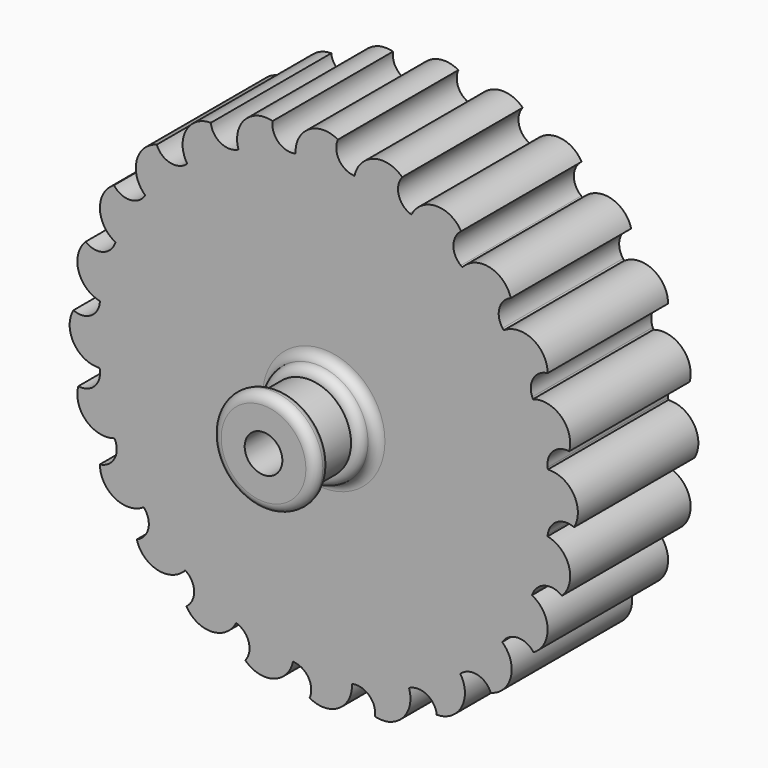
from build123d import *

# Parameters (mm, degrees)
F1_DEPTH     = 50.8
F2_R         = 17.4625
F3_DEPTH     = 6.35
F4_R         = 14.2875
F5_DEPTH     = 12.7
F6_R         = 17.4625
F7_DEPTH     = 6.35
F8_R         = 3.17499
F9_R         = 6.35
F10_DEPTH    = 76.201
F11_T1_DEPTH = 50.8


# Not quite as in the source:
# - a fillet or chamfer that OpenCascade refuses, or shapes differently, is made with other operations: its cross-section is extruded or revolved along the edge and cut away or added
# - a fillet or chamfer is up to 0.001 mm smaller than in the source, because OpenCascade refuses the exact size


with BuildPart() as f1:
    # F0 (on Front) → F1 (new body)
    with BuildSketch(Plane.XZ):
        with BuildLine():
            ThreePointArc((-70.7536357684, 46.348891971), (-75.5114792005, 37.8021981611), (-70.2287691608, 29.5695786604))
            ThreePointArc((-70.2287691608, 29.5695786604), (-72.0845164259, 24.7034914868), (-73.6035479632, 19.7220112368))
            Line((-73.6035479632, 19.7220112368), (-80.338740054, 26.4572033276))
            ThreePointArc((-80.338740054, 26.4572033276), (-82.7224167718, 16.9703105533), (-75.4889519939, 10.3854767276))
            ThreePointArc((-75.4889519939, 10.3854767276), (-76.0220301687, 5.2048947186), (-76.2, 0))
            Line((-76.2, 0), (-84.448891971, 4.7625))
            ThreePointArc((-84.448891971, 4.7625), (-84.2959583455, -5.0180756738), (-75.6046875, -9.5063782813))
            ThreePointArc((-75.6046875, -9.5063782813), (-74.7787681878, -14.6484070232), (-73.6035479632, -19.7220112368))
            Line((-73.6035479632, -19.7220112368), (-82.8039914586, -17.2567598322))
            ThreePointArc((-82.8039914586, -17.2567598322), (-80.1248696635, -26.6644883366), (-70.5680884956, -28.7503893204))
            ThreePointArc((-70.5680884956, -28.7503893204), (-68.4394567327, -33.503444034), (-65.9911357684, -38.1))
            Line((-65.9911357684, -38.1), (-75.5161357684, -38.1))
            ThreePointArc((-75.5161357684, -38.1), (-70.4934035266, -46.4937601844), (-60.7223908795, -46.0351088396))
            ThreePointArc((-60.7223908795, -46.0351088396), (-57.4361094027, -50.075276701), (-53.8815367264, -53.8815367264))
            Line((-53.8815367264, -53.8815367264), (-63.0819802218, -56.346788131))
            ThreePointArc((-63.0819802218, -56.346788131), (-56.0579284352, -63.1545591102), (-46.7385626735, -60.182611768))
            ThreePointArc((-46.7385626735, -60.182611768), (-42.5185861347, -63.234562014), (-38.1, -65.9911357684))
            Line((-38.1, -65.9911357684), (-46.348891971, -70.7536357684))
            ThreePointArc((-46.348891971, -70.7536357684), (-37.8021981611, -75.5114792005), (-29.5695786604, -70.2287691608))
            ThreePointArc((-29.5695786604, -70.2287691608), (-24.7034914868, -72.0845164259), (-19.7220112368, -73.6035479632))
            Line((-19.7220112368, -73.6035479632), (-26.4572033276, -80.338740054))
            ThreePointArc((-26.4572033276, -80.338740054), (-16.9703105533, -82.7224167718), (-10.3854767276, -75.4889519939))
            ThreePointArc((-10.3854767276, -75.4889519939), (-5.2048947186, -76.0220301687), (0, -76.2))
            Line((0, -76.2), (-4.7625, -84.448891971))
            ThreePointArc((-4.7625, -84.448891971), (5.0180756738, -84.2959583455), (9.5063782813, -75.6046875))
            ThreePointArc((9.5063782813, -75.6046875), (14.6484070232, -74.7787681878), (19.7220112368, -73.6035479632))
            Line((19.7220112368, -73.6035479632), (17.2567598322, -82.8039914586))
            ThreePointArc((17.2567598322, -82.8039914586), (26.6644883366, -80.1248696635), (28.7503893204, -70.5680884956))
            ThreePointArc((28.7503893204, -70.5680884956), (33.503444034, -68.4394567327), (38.1, -65.9911357684))
            Line((38.1, -65.9911357684), (38.1, -75.5161357684))
            ThreePointArc((38.1, -75.5161357684), (46.4937601844, -70.4934035266), (46.0351088396, -60.7223908795))
            ThreePointArc((46.0351088396, -60.7223908795), (50.075276701, -57.4361094027), (53.8815367264, -53.8815367264))
            Line((53.8815367264, -53.8815367264), (56.346788131, -63.0819802218))
            ThreePointArc((56.346788131, -63.0819802218), (63.1545591102, -56.0579284352), (60.182611768, -46.7385626735))
            ThreePointArc((60.182611768, -46.7385626735), (63.234562014, -42.5185861347), (65.9911357684, -38.1))
            Line((65.9911357684, -38.1), (70.7536357684, -46.348891971))
            ThreePointArc((70.7536357684, -46.348891971), (75.5114792005, -37.8021981611), (70.2287691608, -29.5695786604))
            ThreePointArc((70.2287691608, -29.5695786604), (72.0845164259, -24.7034914868), (73.6035479632, -19.7220112368))
            Line((73.6035479632, -19.7220112368), (80.338740054, -26.4572033276))
            ThreePointArc((80.338740054, -26.4572033276), (82.7224167718, -16.9703105533), (75.4889519939, -10.3854767276))
            ThreePointArc((75.4889519939, -10.3854767276), (76.0220301687, -5.2048947186), (76.2, 0))
            Line((76.2, 0), (84.448891971, -4.7625))
            ThreePointArc((84.448891971, -4.7625), (84.2959583455, 5.0180756738), (75.6046875, 9.5063782813))
            ThreePointArc((75.6046875, 9.5063782813), (74.7787681878, 14.6484070232), (73.6035479632, 19.7220112368))
            Line((73.6035479632, 19.7220112368), (82.8039914586, 17.2567598322))
            ThreePointArc((82.8039914586, 17.2567598322), (80.1248696635, 26.6644883366), (70.5680884956, 28.7503893204))
            ThreePointArc((70.5680884956, 28.7503893204), (68.4394567327, 33.503444034), (65.9911357684, 38.1))
            Line((65.9911357684, 38.1), (75.5161357684, 38.1))
            ThreePointArc((75.5161357684, 38.1), (70.4934035266, 46.4937601844), (60.7223908795, 46.0351088396))
            ThreePointArc((60.7223908795, 46.0351088396), (57.4361094027, 50.075276701), (53.8815367264, 53.8815367264))
            Line((53.8815367264, 53.8815367264), (63.0819802218, 56.346788131))
            ThreePointArc((63.0819802218, 56.346788131), (56.0579284352, 63.1545591102), (46.7385626735, 60.182611768))
            ThreePointArc((46.7385626735, 60.182611768), (42.5185861347, 63.234562014), (38.1, 65.9911357684))
            Line((38.1, 65.9911357684), (46.348891971, 70.7536357684))
            ThreePointArc((46.348891971, 70.7536357684), (37.8021981611, 75.5114792005), (29.5695786604, 70.2287691608))
            ThreePointArc((29.5695786604, 70.2287691608), (24.7034914868, 72.0845164259), (19.7220112368, 73.6035479632))
            Line((19.7220112368, 73.6035479632), (26.4572033276, 80.338740054))
            ThreePointArc((26.4572033276, 80.338740054), (16.9703105533, 82.7224167718), (10.3854767276, 75.4889519939))
            ThreePointArc((10.3854767276, 75.4889519939), (5.2048947186, 76.0220301687), (0, 76.2))
            Line((0, 76.2), (4.7625, 84.448891971))
            ThreePointArc((4.7625, 84.448891971), (-5.0180756738, 84.2959583455), (-9.5063782813, 75.6046875))
            ThreePointArc((-9.5063782813, 75.6046875), (-14.6484070232, 74.7787681878), (-19.7220112368, 73.6035479632))
            Line((-19.7220112368, 73.6035479632), (-17.2567598322, 82.8039914586))
            ThreePointArc((-17.2567598322, 82.8039914586), (-26.6644883366, 80.1248696635), (-28.7503893204, 70.5680884956))
            ThreePointArc((-28.7503893204, 70.5680884956), (-33.503444034, 68.4394567327), (-38.1, 65.9911357684))
            Line((-38.1, 65.9911357684), (-38.1, 75.5161357684))
            ThreePointArc((-38.1, 75.5161357684), (-46.4937601844, 70.4934035266), (-46.0351088396, 60.7223908795))
            ThreePointArc((-46.0351088396, 60.7223908795), (-50.075276701, 57.4361094027), (-53.8815367264, 53.8815367264))
            Line((-53.8815367264, 53.8815367264), (-56.346788131, 63.0819802218))
            ThreePointArc((-56.346788131, 63.0819802218), (-63.1545591102, 56.0579284352), (-60.182611768, 46.7385626735))
            ThreePointArc((-60.182611768, 46.7385626735), (-63.234562014, 42.5185861347), (-65.9911357684, 38.1))
            Line((-65.9911357684, 38.1), (-70.7536357684, 46.348891971))
        make_face()
    extrude(amount=F1_DEPTH)

    # F2 (on face) → F3 (join)
    with BuildSketch(Plane.XZ.offset(50.8)):
        Circle(F2_R)
    extrude(amount=F3_DEPTH)

    # F4 (on face) → F5 (join)
    with BuildSketch(Plane.XZ.offset(57.15)):
        Circle(F4_R)
    extrude(amount=F5_DEPTH)

    # F6 (on face) → F7 (join)
    with BuildSketch(Plane.XZ.offset(69.85)):
        Circle(F6_R)
    extrude(amount=F7_DEPTH)

    # F8 (radius 3.175 in the source; OpenCascade refuses exactly that, so slightly less here)
    f8_edges = [f1.edges().sort_by_distance(p)[0] for p in [
        (17.4625, -73.025, 0),
        (-17.4625, -69.85, 0),
        (-17.4625, -76.2, 0),
        (17.4625, -53.975, 0),
        (-17.4625, -50.8, 0),
        (-17.4625, -57.15, 0),
    ]]
    fillet(f8_edges, radius=F8_R)

    # F9 (on face) → F10 (cut, through all)
    with BuildSketch(Plane.XZ.offset(76.2)):
        Circle(F9_R)
    extrude(amount=-F10_DEPTH, mode=Mode.SUBTRACT)

    # F11: fillet of radius 6.35 on 24 edges, made by hand

    # F11_s2 → F11_t1 (join)
    with BuildSketch(Plane.XZ):
        with BuildLine():
            ThreePointArc((-46.5419900283, 60.3347591708), (-52.1337249794, 59.2481383586), (-56.346788131, 63.0819802218))
            Line((-56.346788131, 63.0819802218), (-56.4653141097, 63.0363667109))
            ThreePointArc((-56.4653141097, 63.0363667109), (-55.2368350087, 58.4488884554), (-54.0042093064, 53.8486667077))
            Line((-54.0042093064, 53.8486667077), (-53.7917341652, 53.7917341652))
            ThreePointArc((-53.7917341652, 53.7917341652), (-50.2314688194, 57.1305598542), (-46.4644200449, 60.2342012389))
            Line((-46.4644200449, 60.2342012389), (-46.5419900283, 60.3347591708))
        make_face()
        with BuildLine():
            ThreePointArc((-29.3403254202, 70.3248555223), (-35.0227647841, 70.7225079169), (-38.1, 75.5161357684))
            Line((-38.1, 75.5161357684), (-38.2262929492, 75.5027532808))
            ThreePointArc((-38.2262929492, 75.5027532808), (-38.227, 70.7536357684), (-38.227, 65.9911357684))
            Line((-38.227, 65.9911357684), (-38.0365, 65.8811505421))
            ThreePointArc((-38.0365, 65.8811505421), (-33.7333960774, 68.1847440274), (-29.2914248778, 70.2076474298))
            Line((-29.2914248778, 70.2076474298), (-29.3403254202, 70.3248555223))
        make_face()
        with BuildLine():
            ThreePointArc((-17.2567598322, 82.8039914586), (-15.5250610467, 77.3772554351), (-10.1391661218, 75.5224291873))
            Line((-10.1391661218, 75.5224291873), (-10.1222675116, 75.396558472))
            ThreePointArc((-10.1222675116, 75.396558472), (-14.9364481399, 74.5922505758), (-19.6891412181, 73.4808753833))
            Line((-19.6891412181, 73.4808753833), (-19.8446838168, 73.636417982))
            ThreePointArc((-19.8446838168, 73.636417982), (-18.6120581145, 78.2366397297), (-17.3822130962, 82.8237519887))
            Line((-17.3822130962, 82.8237519887), (-17.2567598322, 82.8039914586))
        make_face()
        with BuildLine():
            ThreePointArc((4.7625, 84.448891971), (5.0306499446, 78.7588708674), (9.752960592, 75.5732741099))
            Line((9.752960592, 75.5732741099), (9.7367056577, 75.4473186531))
            ThreePointArc((9.7367056577, 75.4473186531), (4.8783940547, 75.916418517), (0, 76.073))
            Line((0, 76.073), (-0.1099852263, 76.2635))
            ThreePointArc((-0.1099852263, 76.2635), (2.2712647737, 80.3879459855), (4.6464358538, 84.5004488714))
            Line((4.6464358538, 84.5004488714), (4.7625, 84.448891971))
        make_face()
        with BuildLine():
            ThreePointArc((26.4572033276, 80.338740054), (25.2435304558, 74.7731994053), (28.980439159, 70.4739252926))
            Line((28.980439159, 70.4739252926), (28.9321384271, 70.3564687505))
            ThreePointArc((28.9321384271, 70.3564687505), (24.3607817564, 72.0670079941), (19.6891412181, 73.4808753833))
            Line((19.6891412181, 73.4808753833), (19.6322086756, 73.6933505244))
            ThreePointArc((19.6322086756, 73.6933505244), (22.999804721, 77.0609465698), (26.3584378791, 80.4185798071))
            Line((26.3584378791, 80.4185798071), (26.4572033276, 80.338740054))
        make_face()
        with BuildLine():
            ThreePointArc((46.348891971, 70.7536357684), (43.7361060833, 65.6918579723), (46.2329486897, 60.5718949303))
            Line((46.2329486897, 60.5718949303), (46.1558937753, 60.4709417721))
            ThreePointArc((46.1558937753, 60.4709417721), (42.1830224396, 63.3063499727), (38.0365, 65.8811505421))
            Line((38.0365, 65.8811505421), (38.0365, 66.1011209947))
            ThreePointArc((38.0365, 66.1011209947), (42.1609459855, 68.4823709947), (46.2741559222, 70.8563174269))
            Line((46.2741559222, 70.8563174269), (46.348891971, 70.7536357684))
        make_face()
        with BuildLine():
            ThreePointArc((63.0819802218, 56.346788131), (59.2481383586, 52.1337249794), (60.3347591708, 46.5419900283))
            Line((60.3347591708, 46.5419900283), (60.2342012389, 46.4644200449))
            ThreePointArc((60.2342012389, 46.4644200449), (57.1305598542, 50.2314688194), (53.7917341652, 53.7917341652))
            Line((53.7917341652, 53.7917341652), (53.8486667077, 54.0042093064))
            ThreePointArc((53.8486667077, 54.0042093064), (58.4488884554, 55.2368350087), (63.0363667109, 56.4653141097))
            Line((63.0363667109, 56.4653141097), (63.0819802218, 56.346788131))
        make_face()
        with BuildLine():
            ThreePointArc((75.5161357684, 38.1), (70.7225079169, 35.0227647841), (70.3248555223, 29.3403254202))
            Line((70.3248555223, 29.3403254202), (70.2076474298, 29.2914248778))
            ThreePointArc((70.2076474298, 29.2914248778), (68.1847440274, 33.7333960774), (65.8811505421, 38.0365))
            Line((65.8811505421, 38.0365), (65.9911357684, 38.227))
            ThreePointArc((65.9911357684, 38.227), (70.7536357684, 38.227), (75.5027532808, 38.2262929492))
            Line((75.5027532808, 38.2262929492), (75.5161357684, 38.1))
        make_face()
        with BuildLine():
            ThreePointArc((82.8039914586, 17.2567598322), (77.3772554351, 15.5250610467), (75.5224291873, 10.1391661218))
            Line((75.5224291873, 10.1391661218), (75.396558472, 10.1222675116))
            ThreePointArc((75.396558472, 10.1222675116), (74.5922505758, 14.9364481399), (73.4808753833, 19.6891412181))
            Line((73.4808753833, 19.6891412181), (73.636417982, 19.8446838168))
            ThreePointArc((73.636417982, 19.8446838168), (78.2366397297, 18.6120581144), (82.8237519887, 17.3822130962))
            Line((82.8237519887, 17.3822130962), (82.8039914586, 17.2567598322))
        make_face()
        with BuildLine():
            ThreePointArc((84.448891971, -4.7625), (78.7588708674, -5.0306499446), (75.5732741099, -9.752960592))
            Line((75.5732741099, -9.752960592), (75.4473186531, -9.7367056577))
            ThreePointArc((75.4473186531, -9.7367056577), (75.916418517, -4.8783940547), (76.073, 0))
            Line((76.073, 0), (76.2635, 0.1099852263))
            ThreePointArc((76.2635, 0.1099852263), (80.3879459855, -2.2712647737), (84.5004488714, -4.6464358538))
            Line((84.5004488714, -4.6464358538), (84.448891971, -4.7625))
        make_face()
        with BuildLine():
            ThreePointArc((80.338740054, -26.4572033276), (74.7731994053, -25.2435304558), (70.4739252926, -28.980439159))
            Line((70.4739252926, -28.980439159), (70.3564687505, -28.9321384271))
            ThreePointArc((70.3564687505, -28.9321384271), (72.0670079941, -24.3607817564), (73.4808753833, -19.6891412181))
            Line((73.4808753833, -19.6891412181), (73.6933505244, -19.6322086756))
            ThreePointArc((73.6933505244, -19.6322086756), (77.0609465698, -22.999804721), (80.4185798071, -26.3584378791))
            Line((80.4185798071, -26.3584378791), (80.338740054, -26.4572033276))
        make_face()
        with BuildLine():
            ThreePointArc((70.7536357684, -46.348891971), (65.6918579723, -43.7361060833), (60.5718949303, -46.2329486897))
            Line((60.5718949303, -46.2329486897), (60.4709417721, -46.1558937753))
            ThreePointArc((60.4709417721, -46.1558937753), (63.3063499727, -42.1830224396), (65.8811505421, -38.0365))
            Line((65.8811505421, -38.0365), (66.1011209947, -38.0365))
            ThreePointArc((66.1011209947, -38.0365), (68.4823709947, -42.1609459855), (70.8563174269, -46.2741559222))
            Line((70.8563174269, -46.2741559222), (70.7536357684, -46.348891971))
        make_face()
        with BuildLine():
            ThreePointArc((56.346788131, -63.0819802218), (52.1337249794, -59.2481383586), (46.5419900283, -60.3347591708))
            Line((46.5419900283, -60.3347591708), (46.4644200449, -60.2342012389))
            ThreePointArc((46.4644200449, -60.2342012389), (50.2314688194, -57.1305598542), (53.7917341652, -53.7917341652))
            Line((53.7917341652, -53.7917341652), (54.0042093064, -53.8486667077))
            ThreePointArc((54.0042093064, -53.8486667077), (55.2368350087, -58.4488884554), (56.4653141097, -63.0363667109))
            Line((56.4653141097, -63.0363667109), (56.346788131, -63.0819802218))
        make_face()
        with BuildLine():
            ThreePointArc((38.1, -75.5161357684), (35.0227647841, -70.7225079169), (29.3403254202, -70.3248555223))
            Line((29.3403254202, -70.3248555223), (29.2914248778, -70.2076474298))
            ThreePointArc((29.2914248778, -70.2076474298), (33.7333960774, -68.1847440274), (38.0365, -65.8811505421))
            Line((38.0365, -65.8811505421), (38.227, -65.9911357684))
            ThreePointArc((38.227, -65.9911357684), (38.227, -70.7536357684), (38.2262929492, -75.5027532808))
            Line((38.2262929492, -75.5027532808), (38.1, -75.5161357684))
        make_face()
        with BuildLine():
            ThreePointArc((10.1391661218, -75.5224291873), (15.5250610467, -77.3772554351), (17.2567598322, -82.8039914586))
            Line((17.2567598322, -82.8039914586), (17.3822130962, -82.8237519887))
            ThreePointArc((17.3822130962, -82.8237519887), (18.6120581145, -78.2366397297), (19.8446838168, -73.636417982))
            Line((19.8446838168, -73.636417982), (19.6891412181, -73.4808753833))
            ThreePointArc((19.6891412181, -73.4808753833), (14.9364481399, -74.5922505758), (10.1222675116, -75.396558472))
            Line((10.1222675116, -75.396558472), (10.1391661218, -75.5224291873))
        make_face()
        with BuildLine():
            ThreePointArc((-9.752960592, -75.5732741099), (-5.0306499446, -78.7588708674), (-4.7625, -84.448891971))
            Line((-4.7625, -84.448891971), (-4.6464358538, -84.5004488714))
            ThreePointArc((-4.6464358538, -84.5004488714), (-2.2712647737, -80.3879459855), (0.1099852263, -76.2635))
            Line((0.1099852263, -76.2635), (0, -76.073))
            ThreePointArc((0, -76.073), (-4.8783940547, -75.916418517), (-9.7367056577, -75.4473186531))
            Line((-9.7367056577, -75.4473186531), (-9.752960592, -75.5732741099))
        make_face()
        with BuildLine():
            ThreePointArc((-28.980439159, -70.4739252926), (-25.2435304558, -74.7731994053), (-26.4572033276, -80.338740054))
            Line((-26.4572033276, -80.338740054), (-26.3584378791, -80.4185798071))
            ThreePointArc((-26.3584378791, -80.4185798071), (-22.999804721, -77.0609465698), (-19.6322086756, -73.6933505244))
            Line((-19.6322086756, -73.6933505244), (-19.6891412181, -73.4808753833))
            ThreePointArc((-19.6891412181, -73.4808753833), (-24.3607817564, -72.0670079941), (-28.9321384271, -70.3564687505))
            Line((-28.9321384271, -70.3564687505), (-28.980439159, -70.4739252926))
        make_face()
        with BuildLine():
            ThreePointArc((-46.2329486897, -60.5718949303), (-43.7361060833, -65.6918579723), (-46.348891971, -70.7536357684))
            Line((-46.348891971, -70.7536357684), (-46.2741559222, -70.8563174269))
            ThreePointArc((-46.2741559222, -70.8563174269), (-42.1609459855, -68.4823709947), (-38.0365, -66.1011209947))
            Line((-38.0365, -66.1011209947), (-38.0365, -65.8811505421))
            ThreePointArc((-38.0365, -65.8811505421), (-42.1830224396, -63.3063499727), (-46.1558937753, -60.4709417721))
            Line((-46.1558937753, -60.4709417721), (-46.2329486897, -60.5718949303))
        make_face()
        with BuildLine():
            ThreePointArc((-60.3347591708, -46.5419900283), (-59.2481383586, -52.1337249794), (-63.0819802218, -56.346788131))
            Line((-63.0819802218, -56.346788131), (-63.0363667109, -56.4653141097))
            ThreePointArc((-63.0363667109, -56.4653141097), (-58.4488884554, -55.2368350087), (-53.8486667077, -54.0042093064))
            Line((-53.8486667077, -54.0042093064), (-53.7917341652, -53.7917341652))
            ThreePointArc((-53.7917341652, -53.7917341652), (-57.1305598542, -50.2314688194), (-60.2342012389, -46.4644200449))
            Line((-60.2342012389, -46.4644200449), (-60.3347591708, -46.5419900283))
        make_face()
        with BuildLine():
            ThreePointArc((-70.3248555223, -29.3403254202), (-70.7225079169, -35.0227647841), (-75.5161357684, -38.1))
            Line((-75.5161357684, -38.1), (-75.5027532808, -38.2262929492))
            ThreePointArc((-75.5027532808, -38.2262929492), (-70.7536357684, -38.227), (-65.9911357684, -38.227))
            Line((-65.9911357684, -38.227), (-65.8811505421, -38.0365))
            ThreePointArc((-65.8811505421, -38.0365), (-68.1847440274, -33.7333960774), (-70.2076474298, -29.2914248778))
            Line((-70.2076474298, -29.2914248778), (-70.3248555223, -29.3403254202))
        make_face()
        with BuildLine():
            ThreePointArc((-75.5224291873, -10.1391661218), (-77.3772554351, -15.5250610467), (-82.8039914586, -17.2567598322))
            Line((-82.8039914586, -17.2567598322), (-82.8237519887, -17.3822130962))
            ThreePointArc((-82.8237519887, -17.3822130962), (-78.2366397297, -18.6120581145), (-73.636417982, -19.8446838168))
            Line((-73.636417982, -19.8446838168), (-73.4808753833, -19.6891412181))
            ThreePointArc((-73.4808753833, -19.6891412181), (-74.5922505758, -14.9364481399), (-75.396558472, -10.1222675116))
            Line((-75.396558472, -10.1222675116), (-75.5224291873, -10.1391661218))
        make_face()
        with BuildLine():
            ThreePointArc((-75.5732741099, 9.752960592), (-78.7588708674, 5.0306499446), (-84.448891971, 4.7625))
            Line((-84.448891971, 4.7625), (-84.5004488714, 4.6464358538))
            ThreePointArc((-84.5004488714, 4.6464358538), (-80.3879459855, 2.2712647737), (-76.2635, -0.1099852263))
            Line((-76.2635, -0.1099852263), (-76.073, 0))
            ThreePointArc((-76.073, 0), (-75.916418517, 4.8783940547), (-75.4473186531, 9.7367056577))
            Line((-75.4473186531, 9.7367056577), (-75.5732741099, 9.752960592))
        make_face()
        with BuildLine():
            ThreePointArc((-70.4739252926, 28.980439159), (-74.7731994053, 25.2435304558), (-80.338740054, 26.4572033276))
            Line((-80.338740054, 26.4572033276), (-80.4185798071, 26.3584378791))
            ThreePointArc((-80.4185798071, 26.3584378791), (-77.0609465698, 22.999804721), (-73.6933505244, 19.6322086756))
            Line((-73.6933505244, 19.6322086756), (-73.4808753833, 19.6891412181))
            ThreePointArc((-73.4808753833, 19.6891412181), (-72.0670079941, 24.3607817564), (-70.3564687505, 28.9321384271))
            Line((-70.3564687505, 28.9321384271), (-70.4739252926, 28.980439159))
        make_face()
        with BuildLine():
            ThreePointArc((-60.5718949303, 46.2329486897), (-65.6918579723, 43.7361060833), (-70.7536357684, 46.348891971))
            Line((-70.7536357684, 46.348891971), (-70.8563174269, 46.2741559222))
            ThreePointArc((-70.8563174269, 46.2741559222), (-68.4823709947, 42.1609459855), (-66.1011209947, 38.0365))
            Line((-66.1011209947, 38.0365), (-65.8811505421, 38.0365))
            ThreePointArc((-65.8811505421, 38.0365), (-63.3063499727, 42.1830224396), (-60.4709417721, 46.1558937753))
            Line((-60.4709417721, 46.1558937753), (-60.5718949303, 46.2329486897))
        make_face()
    extrude(amount=F11_T1_DEPTH)


solid = f1.part
